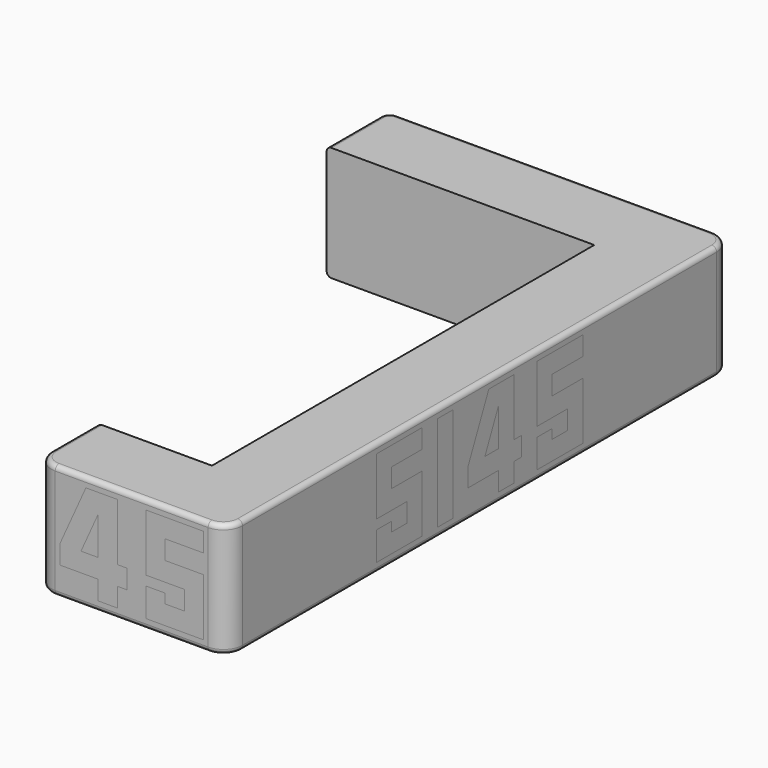
from build123d import *

# Parameters (mm, degrees)
F1_DEPTH  = 152.4
F2_R      = 25.4
F3_W      = 25.4
F3_H      = 127
F4_DEPTH  = 25.4
F5_DEPTH  = 25.4
F7_DEPTH  = 25.4
F8_DEPTH  = 25.4
F9_W      = 25.4
F9_H      = 127
F10_DEPTH = 25.4
F11_DEPTH = 25.4
F12_R     = 12.69999
F13_R     = 6.35


# Not quite as in the source:
# - a fillet or chamfer is up to 0.001 mm smaller than in the source, because OpenCascade refuses the exact size


with BuildPart() as f1:
    # F0 (on Top) → F1 (new body)
    with BuildSketch(Plane.XY):
        Polygon((-261.3841307829, 381.0432040095), (-261.3841307829, 279.4432040095), (94.2158692171, 279.4432040095), (94.2158692171, -355.5567959905), (-58.1841307829, -355.5567959905), (-58.1841307829, -457.1567959905), (195.8158692171, -457.1567959905), (195.8158692171, 381.0432040095), align=None)
    extrude(amount=F1_DEPTH)

    # F2
    f2_edges = [f1.edges().sort_by_distance(p)[0] for p in [
        (195.815869, -457.156796, 76.2),
        (-58.184131, -457.156796, 76.2),
        (195.815869, 381.043204, 76.2),
    ]]
    fillet(f2_edges, radius=F2_R)

    # F3 (on face) → F4 (cut)
    with BuildSketch(Plane.YZ.offset(195.8158692171)):
        Polygon((-133.3067959905, 114.3), (-133.3067959905, 139.7), (-209.5067959905, 139.7), (-209.5067959905, 63.5), (-158.7067959905, 63.5), (-158.7067959905, 38.1), (-184.1067959905, 38.1), (-184.1067959905, 50.8), (-209.5067959905, 50.8), (-209.5067959905, 12.7), (-133.3067959905, 12.7), (-133.3067959905, 88.9), (-184.1067959905, 88.9), (-184.1067959905, 114.3), align=None)
        with Locations((-95.2067959905, 76.2)):
            Rectangle(F3_W, F3_H)
        Polygon((19.0932040095, 63.5), (19.0932040095, 139.7), (-22.7088792915, 139.7), (-57.1067959905, 63.5), (-57.1067959905, 38.1), (-6.3067959905, 38.1), (-6.3067959905, 12.7), (19.0932040095, 12.7), (19.0932040095, 38.1), (31.7932040095, 38.1), (31.7932040095, 63.5), align=None)
        Polygon((-6.3067959905, 114.3), (-6.3067959905, 63.5), (-29.2387404565, 63.5), align=None, mode=Mode.SUBTRACT)
        Polygon((133.3932040095, 114.3), (133.3932040095, 139.7), (57.1932040095, 139.7), (57.1932040095, 63.5), (107.9932040095, 63.5), (107.9932040095, 38.1), (82.5932040095, 38.1), (82.5932040095, 50.8), (57.1932040095, 50.8), (57.1932040095, 12.7), (133.3932040095, 12.7), (133.3932040095, 88.9), (82.5932040095, 88.9), (82.5932040095, 114.3), align=None)
    extrude(amount=-F4_DEPTH, mode=Mode.SUBTRACT)


with BuildPart() as f5:
    # F5 (new): a face of the model
    f5_faces = [f1.part.faces().sort_by_distance(p)[0] for p in [
        (170.4158692171, -172.5111438166, 74.8195652174),
    ]]
    extrude(f5_faces, amount=F5_DEPTH)


with BuildPart() as f5b:
    # F5#2 (new): a face of the model
    f5_2_faces = [f1.part.faces().sort_by_distance(p)[0] for p in [
        (170.4158692171, -95.2067959905, 76.2),
    ]]
    extrude(f5_2_faces, amount=F5_DEPTH)


with BuildPart() as f5c:
    # F5#3 (new): a face of the model
    f5_3_faces = [f1.part.faces().sort_by_distance(p)[0] for p in [
        (170.4158692171, 25.4432040095, 61.9497674368),
    ]]
    extrude(f5_3_faces, amount=F5_DEPTH)


with BuildPart() as f5d:
    # F5#4 (new): a face of the model
    f5_4_faces = [f1.part.faces().sort_by_distance(p)[0] for p in [
        (170.4158692171, 94.1888561834, 74.8195652174),
    ]]
    extrude(f5_4_faces, amount=F5_DEPTH)


with BuildPart() as f1_1:
    add(f1.part)

    # F6 (on face) → F7 (cut)
    with BuildSketch(Plane.XZ.offset(457.1567959905)):
        Polygon((49.7658692171, 139.7), (7.9637859161, 139.7), (-26.4341307829, 63.5), (-26.4341307829, 38.1), (24.3658692171, 38.1), (24.3658692171, 12.7), (49.7658692171, 12.7), (49.7658692171, 38.1), (62.4658692171, 38.1), (62.4658692171, 63.5), (49.7658692171, 63.5), align=None)
        Polygon((24.3658692171, 114.3), (24.3658692171, 63.5), (1.4339247512, 63.5), align=None, mode=Mode.SUBTRACT)
        Polygon((164.0658692171, 114.3), (164.0658692171, 139.7), (87.8658692171, 139.7), (87.8658692171, 63.5), (138.6658692171, 63.5), (138.6658692171, 38.1), (113.2658692171, 38.1), (113.2658692171, 50.8), (87.8658692171, 50.8), (87.8658692171, 12.7), (164.0658692171, 12.7), (164.0658692171, 88.9), (113.2658692171, 88.9), (113.2658692171, 114.3), align=None)
    extrude(amount=-F7_DEPTH, mode=Mode.SUBTRACT)


with BuildPart() as f8:
    # F8 (new): a face of the model
    f8_faces = [f1_1.part.faces().sort_by_distance(p)[0] for p in [
        (48.2156366539, -431.7567959905, 101.6),
    ]]
    extrude(f8_faces, amount=F8_DEPTH)


with BuildPart() as f8b:
    # F8#2 (new): a face of the model
    f8_2_faces = [f1_1.part.faces().sort_by_distance(p)[0] for p in [
        (124.8615213911, -431.7567959905, 74.8195652174),
    ]]
    extrude(f8_2_faces, amount=F8_DEPTH)


with BuildPart() as f1_2:
    add(f1_1.part)

    # F9 (on face) → F10 (cut)
    with BuildSketch(Plane(origin=(0, 381.0432040095, 0), x_dir=(-1, 0, 0), z_dir=(0, 1, 0))):
        Polygon((197.8841307829, 114.3), (197.8841307829, 139.7), (121.6841307829, 139.7), (121.6841307829, 63.5), (172.4841307829, 63.5), (172.4841307829, 38.1), (147.0841307829, 38.1), (147.0841307829, 50.8), (121.6841307829, 50.8), (121.6841307829, 12.7), (197.8841307829, 12.7), (197.8841307829, 88.9), (147.0841307829, 88.9), (147.0841307829, 114.3), align=None)
        with Locations((235.9841307829, 76.2)):
            Rectangle(F9_W, F9_H)
    extrude(amount=-F10_DEPTH, mode=Mode.SUBTRACT)


with BuildPart() as f11:
    # F11 (new): a face of the model
    f11_faces = [f1_2.part.faces().sort_by_distance(p)[0] for p in [
        (-158.6797829568, 355.6432040095, 74.8195652174),
    ]]
    extrude(f11_faces, amount=F11_DEPTH)


with BuildPart() as f11b:
    # F11#2 (new): a face of the model
    f11_2_faces = [f1_2.part.faces().sort_by_distance(p)[0] for p in [
        (-235.9841307829, 355.6432040095, 76.2),
    ]]
    extrude(f11_2_faces, amount=F11_DEPTH)


with BuildPart() as f1_3:
    add(f1_2.part)

    # F12 (radius 12.7 in the source; OpenCascade refuses exactly that, so slightly less here)
    f12_edges = [f1_3.edges().sort_by_distance(p)[0] for p in [
        (-261.384131, 381.043204, 76.2),
    ]]
    fillet(f12_edges, radius=F12_R)

    # F13
    f13_edges = [f1_3.edges().sort_by_distance(p)[0] for p in [
        (68.815869, -457.156796, 152.4),
        (195.815869, -38.056796, 0),
    ]]
    fillet(f13_edges, radius=F13_R)


solid = Compound([f5.part, f5b.part, f5c.part, f5d.part, f8.part, f8b.part, f11.part, f11b.part, f1_3.part])
